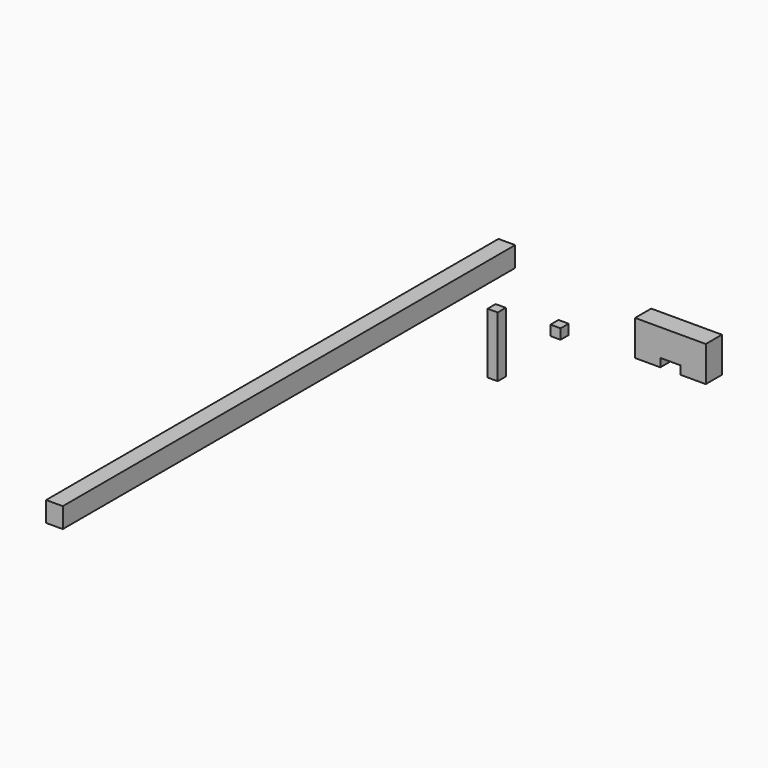
from build123d import *

# Parameters (mm, degrees)
F1_DEPTH = 50.8
F0_W     = 42
F0_H     = 50.8
F2_DEPTH = 1422.4
F0_W_2   = 25.4
F0_H_2   = 25.4
F3_DEPTH = 25.4
F0_H_3   = 152.4


# Not quite as in the source:
# - a feature names something its author has since deleted; it is built from what else it names


with BuildPart() as f1:
    # F0 (on Front) → F1 (new body)
    with BuildSketch(Plane.XZ):
        Polygon((472.1291068077, 21.6997341752), (294.3291068077, 21.6997341752), (294.3291068077, -67.2002658248), (357.8291068077, -67.2002658248), (357.8291068077, -46.2002658248), (408.6291068077, -46.2002658248), (408.6291068077, -67.2002658248), (472.1291068077, -67.2002658248), align=None)
    extrude(amount=F1_DEPTH)


with BuildPart() as f2:
    # F0 (on Front) → F2 (new body)
    with BuildSketch(Plane.XZ):
        with Locations((-68.8863479115, 25.6433247801)):
            Rectangle(F0_W, F0_H)
    extrude(amount=F2_DEPTH)


with BuildPart() as f3:
    # F0 (on Front) → F3 (new body)
    with BuildSketch(Plane.XZ):
        with Locations((73.7957331955, -92.0277962789)):
            Rectangle(F0_W_2, F0_H_2)
    extrude(amount=F3_DEPTH)


with BuildPart() as f3b:
    # F0 (on Front) → F3, piece 2 (new body)
    with BuildSketch(Plane.XZ):
        with Locations((-84.2424545765, -171.7660920799)):
            Rectangle(F0_W_2, F0_H_3)
    extrude(amount=F3_DEPTH)


solid = Compound([f1.part, f2.part, f3.part, f3b.part])
